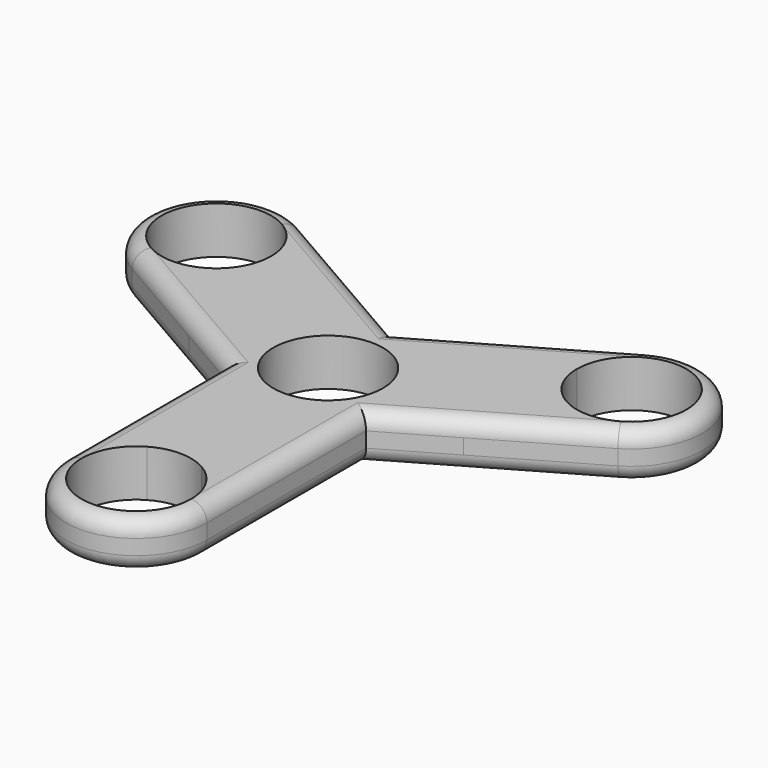
from build123d import *

# Parameters (mm, degrees)
F0_R          = 3.5
F1_DEPTH      = 3
F2_T4_DEPTH   = 15.24
F2_T9_DEPTH   = 15.24
F2_T14_DEPTH  = 15.24
F2_T19_DEPTH  = 15.24
F2_T24_DEPTH  = 15.24
F2_T29_DEPTH  = 15.24
F2_T32_ANGLE  = 180
F2_T34_ANGLE  = 180
F2_T36_ANGLE  = 180
F2_T40_DEPTH  = 15.24
F2_T45_DEPTH  = 15.24
F2_T50_DEPTH  = 15.24
F2_T55_DEPTH  = 15.24
F2_T58_ANGLE  = 180
F2_T62_DEPTH  = 15.24
F2_T65_ANGLE  = 180
F2_T67_ANGLE  = 180
F2_T71_DEPTH  = 15.24
F2_T77_DEPTH  = 15.24
F2_T81_DEPTH  = 15.24
F2_T88_DEPTH  = 15.24
F2_T92_DEPTH  = 15.24
F2_T99_DEPTH  = 15.24
F2_T103_DEPTH = 15.24
F2_T110_DEPTH = 15.24
F2_T114_DEPTH = 15.24
F2_T121_DEPTH = 15.24
F2_T125_DEPTH = 15.24
F2_T132_DEPTH = 15.24
F2_T136_DEPTH = 15.24


# Not quite as in the source:
# - a fillet or chamfer that OpenCascade refuses, or shapes differently, is made with other operations: its cross-section is extruded or revolved along the edge and cut away or added


with BuildPart() as f1:
    # F0 (on Top) → F1 (new body)
    with BuildSketch(Plane.XY):
        with BuildLine():
            Line((-9.7485226281, 10.247114317), (-8.7485226281, 10.247114317))
            ThreePointArc((-8.7485226281, 10.247114317), (-9.351408311, 12.497114317), (-10.9985226281, 14.1442286341))
            ThreePointArc((-10.9985226281, 14.1442286341), (-17.1456369451, 12.497114317), (-15.4985226281, 6.35))
            ThreePointArc((-15.4985226281, 6.35), (-13.2485226281, 5.747114317), (-10.9985226281, 6.35))
            Line((-10.9985226281, 6.35), (-11.4985226281, 7.2160254038))
            ThreePointArc((-11.4985226281, 7.2160254038), (-16.2796115413, 11.997114317), (-9.7485226281, 10.247114317))
        make_face()
        with BuildLine():
            ThreePointArc((-10.9985226281, 6.35), (-9.351408311, 7.997114317), (-8.7485226281, 10.247114317))
            Line((-8.7485226281, 10.247114317), (-9.7485226281, 10.247114317))
            ThreePointArc((-9.7485226281, 10.247114317), (-10.2174337148, 8.497114317), (-11.4985226281, 7.2160254038))
            Line((-11.4985226281, 7.2160254038), (-10.9985226281, 6.35))
        make_face()
        with BuildLine():
            Line((9.7485226281, 10.247114317), (8.7485226281, 10.247114317))
            ThreePointArc((8.7485226281, 10.247114317), (9.351408311, 7.997114317), (10.9985226281, 6.35))
            Line((10.9985226281, 6.35), (11.4985226281, 7.2160254038))
            ThreePointArc((11.4985226281, 7.2160254038), (10.2174337148, 8.497114317), (9.7485226281, 10.247114317))
        make_face()
        with BuildLine():
            ThreePointArc((17.7485226281, 10.247114317), (15.4985226281, 14.1442286341), (10.9985226281, 14.1442286341))
            ThreePointArc((10.9985226281, 14.1442286341), (9.351408311, 12.497114317), (8.7485226281, 10.247114317))
            Line((8.7485226281, 10.247114317), (9.7485226281, 10.247114317))
            ThreePointArc((9.7485226281, 10.247114317), (13.2485226281, 13.747114317), (16.7485226281, 10.247114317))
            ThreePointArc((16.7485226281, 10.247114317), (14.9985226281, 7.2160254038), (11.4985226281, 7.2160254038))
            Line((11.4985226281, 7.2160254038), (10.9985226281, 6.35))
            ThreePointArc((10.9985226281, 6.35), (13.2485226281, 5.747114317), (15.4985226281, 6.35))
            ThreePointArc((15.4985226281, 6.35), (17.1456369451, 7.997114317), (17.7485226281, 10.247114317))
        make_face()
        with BuildLine():
            ThreePointArc((2.25, -8.802885683), (0, -8.2), (-2.25, -8.802885683))
            Line((-2.25, -8.802885683), (-1.75, -9.6689110868))
            ThreePointArc((-1.75, -9.6689110868), (0, -9.2), (1.75, -9.6689110868))
            Line((1.75, -9.6689110868), (2.25, -8.802885683))
        make_face()
        with BuildLine():
            ThreePointArc((-2.25, -8.802885683), (-3.897114317, -10.45), (-4.5, -12.7))
            ThreePointArc((-4.5, -12.7), (0, -17.2), (4.5, -12.7))
            ThreePointArc((4.5, -12.7), (3.897114317, -10.45), (2.25, -8.802885683))
            Line((2.25, -8.802885683), (1.75, -9.6689110868))
            ThreePointArc((1.75, -9.6689110868), (3.0310889132, -10.95), (3.5, -12.7))
            ThreePointArc((3.5, -12.7), (-1.75, -15.7310889132), (-1.75, -9.6689110868))
            Line((-1.75, -9.6689110868), (-2.25, -8.802885683))
        make_face()
        with BuildLine():
            Line((-4.2485226281, 10.247114317), (-8.7485226281, 10.247114317))
            ThreePointArc((-8.7485226281, 10.247114317), (-9.351408311, 7.997114317), (-10.9985226281, 6.35))
            Line((-10.9985226281, 6.35), (-8.7485226281, 2.452885683))
            Line((-8.7485226281, 2.452885683), (-4.5, 0))
            Line((-4.5, 0), (-4.5, -4.9057713659))
            Line((-4.5, -4.9057713659), (-2.25, -8.802885683))
            ThreePointArc((-2.25, -8.802885683), (0, -8.2), (2.25, -8.802885683))
            Line((2.25, -8.802885683), (4.5, -4.9057713659))
            Line((4.5, -4.9057713659), (4.5, 0))
            Line((4.5, 0), (8.7485226281, 2.452885683))
            Line((8.7485226281, 2.452885683), (10.9985226281, 6.35))
            ThreePointArc((10.9985226281, 6.35), (9.351408311, 7.997114317), (8.7485226281, 10.247114317))
            Line((8.7485226281, 10.247114317), (4.2485226281, 10.247114317))
            Line((4.2485226281, 10.247114317), (0, 7.7942286341))
            Line((0, 7.7942286341), (-4.2485226281, 10.247114317))
        make_face()
        with Locations((0, 2.5980762114)):
            Circle(F0_R, mode=Mode.SUBTRACT)
        with BuildLine():
            Line((-2.25, -8.802885683), (-4.5, -4.9057713659))
            Line((-4.5, -4.9057713659), (-4.5, -12.7))
            ThreePointArc((-4.5, -12.7), (-3.897114317, -10.45), (-2.25, -8.802885683))
        make_face()
        with BuildLine():
            ThreePointArc((2.25, -8.802885683), (3.897114317, -10.45), (4.5, -12.7))
            Line((4.5, -12.7), (4.5, -4.9057713659))
            Line((4.5, -4.9057713659), (2.25, -8.802885683))
        make_face()
        with BuildLine():
            ThreePointArc((15.4985226281, 6.35), (13.2485226281, 5.747114317), (10.9985226281, 6.35))
            Line((10.9985226281, 6.35), (8.7485226281, 2.452885683))
            Line((8.7485226281, 2.452885683), (15.4985226281, 6.35))
        make_face()
        with BuildLine():
            Line((10.9985226281, 14.1442286341), (4.2485226281, 10.247114317))
            Line((4.2485226281, 10.247114317), (8.7485226281, 10.247114317))
            ThreePointArc((8.7485226281, 10.247114317), (9.351408311, 12.497114317), (10.9985226281, 14.1442286341))
        make_face()
        with BuildLine():
            ThreePointArc((-10.9985226281, 14.1442286341), (-9.351408311, 12.497114317), (-8.7485226281, 10.247114317))
            Line((-8.7485226281, 10.247114317), (-4.2485226281, 10.247114317))
            Line((-4.2485226281, 10.247114317), (-10.9985226281, 14.1442286341))
        make_face()
        with BuildLine():
            Line((-8.7485226281, 2.452885683), (-10.9985226281, 6.35))
            ThreePointArc((-10.9985226281, 6.35), (-13.2485226281, 5.747114317), (-15.4985226281, 6.35))
            Line((-15.4985226281, 6.35), (-8.7485226281, 2.452885683))
        make_face()
    extrude(amount=F1_DEPTH)

    # F2: fillet of radius 1.016 on 18 edges, made by hand


with BuildPart() as f2_tool2:
    # F2_s3 → F2_t4 (new body)
    with BuildSketch(Plane(origin=(14.3735226281, 8.2985571585, 0), x_dir=(0, 0, 1), z_dir=(-0.8660254038, -0.5, 0))):
        with BuildLine():
            ThreePointArc((1.984, 6.75), (2.7024204897, 6.4524204897), (3, 5.734))
            Line((3, 5.734), (3, 6.75))
            Line((3, 6.75), (1.984, 6.75))
        make_face()
    extrude(amount=F2_T4_DEPTH)

    split(bisect_by=Plane(origin=(3.375, 5.8456714755, 0), x_dir=(0, 0, 1), z_dir=(0.5, 0.8660254038, 0)), keep=Keep.TOP)


with BuildPart() as f1_1:
    add(f1.part)

    # F2_t1: cut F2_tool2
    add(f2_tool2.part, mode=Mode.SUBTRACT)


with BuildPart() as f2_tool7:
    # F2_s8 → F2_t9 (new body)
    with BuildSketch(Plane(origin=(1.1752954744, 0.6785571585, 0), x_dir=(0, 0, 1), z_dir=(0.8660254038, 0.5, 0))):
        with BuildLine():
            ThreePointArc((1.984, 2.25), (2.7024204897, 1.9524204897), (3, 1.234))
            Line((3, 1.234), (3, 2.25))
            Line((3, 2.25), (1.984, 2.25))
        make_face()
    extrude(amount=F2_T9_DEPTH)

    split(bisect_by=Plane.YZ.offset(4.5), keep=Keep.TOP)


with BuildPart() as f1_2:
    add(f1_1.part)

    # F2_t6: cut F2_tool7
    add(f2_tool7.part, mode=Mode.SUBTRACT)


with BuildPart() as f2_tool12:
    # F2_s13 → F2_t14 (new body)
    with BuildSketch(Plane(origin=(-1.1752954744, 0.6785571585, 0), x_dir=(0, 0, 1), z_dir=(-0.8660254038, 0.5, 0))):
        with BuildLine():
            ThreePointArc((1.984, 6.75), (2.7024204897, 6.4524204897), (3, 5.734))
            Line((3, 5.734), (3, 6.75))
            Line((3, 6.75), (1.984, 6.75))
        make_face()
    extrude(amount=F2_T14_DEPTH)

    split(bisect_by=Plane(origin=(-3.375, 5.8456714755, 0), x_dir=(0, 0, 1), z_dir=(-0.5, 0.8660254038, 0)), keep=Keep.TOP)


with BuildPart() as f1_3:
    add(f1_2.part)

    # F2_t11: cut F2_tool12
    add(f2_tool12.part, mode=Mode.SUBTRACT)


with BuildPart() as f2_tool17:
    # F2_s18 → F2_t19 (new body)
    with BuildSketch(Plane(origin=(-14.3735226281, 8.2985571585, 0), x_dir=(0, 0, 1), z_dir=(0.8660254038, -0.5, 0))):
        with BuildLine():
            ThreePointArc((1.984, 2.25), (2.7024204897, 1.9524204897), (3, 1.234))
            Line((3, 1.234), (3, 2.25))
            Line((3, 2.25), (1.984, 2.25))
        make_face()
    extrude(amount=F2_T19_DEPTH)

    split(bisect_by=Plane.YZ.offset(-4.5), keep=Keep.BOTTOM)


with BuildPart() as f1_4:
    add(f1_3.part)

    # F2_t16: cut F2_tool17
    add(f2_tool17.part, mode=Mode.SUBTRACT)


with BuildPart() as f2_tool22:
    # F2_s23 → F2_t24 (new body)
    with BuildSketch(Plane.XZ.offset(-2.54)):
        with BuildLine():
            ThreePointArc((-4.5, 1.984), (-4.2024204897, 2.7024204897), (-3.484, 3))
            Line((-3.484, 3), (-4.5, 3))
            Line((-4.5, 3), (-4.5, 1.984))
        make_face()
    extrude(amount=F2_T24_DEPTH)

    split(bisect_by=Plane(origin=(-1.125, -1.9485571585, 0), x_dir=(0, 0, 1), z_dir=(-0.5, -0.8660254038, 0)), keep=Keep.TOP)


with BuildPart() as f1_5:
    add(f1_4.part)

    # F2_t21: cut F2_tool22
    add(f2_tool22.part, mode=Mode.SUBTRACT)


with BuildPart() as f2_tool27:
    # F2_s28 → F2_t29 (new body)
    with BuildSketch(Plane.XZ.offset(12.7)):
        with BuildLine():
            ThreePointArc((4.5, 1.984), (4.2024204897, 2.7024204897), (3.484, 3))
            Line((3.484, 3), (4.5, 3))
            Line((4.5, 3), (4.5, 1.984))
        make_face()
    extrude(amount=-F2_T29_DEPTH)

    split(bisect_by=Plane(origin=(1.125, -1.9485571585, 0), x_dir=(0, 0, 1), z_dir=(0.5, -0.8660254038, 0)), keep=Keep.TOP)


with BuildPart() as f1_6:
    add(f1_5.part)

    # F2_t26: cut F2_tool27
    add(f2_tool27.part, mode=Mode.SUBTRACT)

    # F2_s31 → F2_t32 (revolve, cut)
    with BuildSketch(Plane.XZ.offset(12.7)):
        with BuildLine():
            ThreePointArc((-4.5, 1.984), (-4.2024204897, 2.7024204897), (-3.484, 3))
            Line((-3.484, 3), (-4.5, 3))
            Line((-4.5, 3), (-4.5, 1.984))
        make_face()
    revolve(axis=Axis((0, -12.7, 3), (0, 0, 1)), revolution_arc=F2_T32_ANGLE, mode=Mode.SUBTRACT)

    # F2_s33 → F2_t34 (revolve, cut)
    with BuildSketch(Plane(origin=(-14.3735226281, 8.2985571585, 0), x_dir=(0, 0, 1), z_dir=(0.8660254038, -0.5, 0))):
        with BuildLine():
            ThreePointArc((1.984, -6.75), (2.7024204897, -6.4524204897), (3, -5.734))
            Line((3, -5.734), (3, -6.75))
            Line((3, -6.75), (1.984, -6.75))
        make_face()
    revolve(axis=Axis((-13.2485226281, 10.247114317, 3), (0, 0, 1)), revolution_arc=F2_T34_ANGLE, mode=Mode.SUBTRACT)

    # F2_s35 → F2_t36 (revolve, cut)
    with BuildSketch(Plane(origin=(14.3735226281, 8.2985571585, 0), x_dir=(0, 0, 1), z_dir=(-0.8660254038, -0.5, 0))):
        with BuildLine():
            ThreePointArc((1.984, -2.25), (2.7024204897, -1.9524204897), (3, -1.234))
            Line((3, -1.234), (3, -2.25))
            Line((3, -2.25), (1.984, -2.25))
        make_face()
    revolve(axis=Axis((13.2485226281, 10.247114317, 3), (0, 0, 1)), revolution_arc=F2_T36_ANGLE, mode=Mode.SUBTRACT)


with BuildPart() as f2_tool38:
    # F2_s39 → F2_t40 (new body)
    with BuildSketch(Plane(origin=(-14.3735226281, 8.2985571585, 0), x_dir=(0, 0, 1), z_dir=(0.8660254038, -0.5, 0))):
        with BuildLine():
            ThreePointArc((1.016, 2.25), (0.2975795103, 1.9524204897), (0, 1.234))
            Line((0, 1.234), (0, 2.25))
            Line((0, 2.25), (1.016, 2.25))
        make_face()
    extrude(amount=F2_T40_DEPTH)

    split(bisect_by=Plane.YZ.offset(-4.5), keep=Keep.BOTTOM)


with BuildPart() as f1_7:
    add(f1_6.part)

    # F2_t37: cut F2_tool38
    add(f2_tool38.part, mode=Mode.SUBTRACT)


with BuildPart() as f2_tool43:
    # F2_s44 → F2_t45 (new body)
    with BuildSketch(Plane.XZ.offset(-2.54)):
        with BuildLine():
            ThreePointArc((-4.5, 1.016), (-4.2024204897, 0.2975795103), (-3.484, 0))
            Line((-3.484, 0), (-4.5, 0))
            Line((-4.5, 0), (-4.5, 1.016))
        make_face()
    extrude(amount=F2_T45_DEPTH)

    split(bisect_by=Plane(origin=(-1.125, -1.9485571585, 0), x_dir=(0, 0, 1), z_dir=(-0.5, -0.8660254038, 0)), keep=Keep.TOP)


with BuildPart() as f1_8:
    add(f1_7.part)

    # F2_t42: cut F2_tool43
    add(f2_tool43.part, mode=Mode.SUBTRACT)


with BuildPart() as f2_tool48:
    # F2_s49 → F2_t50 (new body)
    with BuildSketch(Plane.XZ.offset(12.7)):
        with BuildLine():
            ThreePointArc((4.5, 1.016), (4.2024204897, 0.2975795103), (3.484, 0))
            Line((3.484, 0), (4.5, 0))
            Line((4.5, 0), (4.5, 1.016))
        make_face()
    extrude(amount=-F2_T50_DEPTH)

    split(bisect_by=Plane(origin=(1.125, -1.9485571585, 0), x_dir=(0, 0, 1), z_dir=(0.5, -0.8660254038, 0)), keep=Keep.TOP)


with BuildPart() as f1_9:
    add(f1_8.part)

    # F2_t47: cut F2_tool48
    add(f2_tool48.part, mode=Mode.SUBTRACT)


with BuildPart() as f2_tool53:
    # F2_s54 → F2_t55 (new body)
    with BuildSketch(Plane(origin=(1.1752954744, 0.6785571585, 0), x_dir=(0, 0, 1), z_dir=(0.8660254038, 0.5, 0))):
        with BuildLine():
            ThreePointArc((1.016, 2.25), (0.2975795103, 1.9524204897), (0, 1.234))
            Line((0, 1.234), (0, 2.25))
            Line((0, 2.25), (1.016, 2.25))
        make_face()
    extrude(amount=F2_T55_DEPTH)

    split(bisect_by=Plane.YZ.offset(4.5), keep=Keep.TOP)


with BuildPart() as f1_10:
    add(f1_9.part)

    # F2_t52: cut F2_tool53
    add(f2_tool53.part, mode=Mode.SUBTRACT)

    # F2_s57 → F2_t58 (revolve, cut)
    with BuildSketch(Plane(origin=(14.3735226281, 8.2985571585, 0), x_dir=(0, 0, 1), z_dir=(-0.8660254038, -0.5, 0))):
        with BuildLine():
            ThreePointArc((1.016, -2.25), (0.2975795103, -1.9524204897), (0, -1.234))
            Line((0, -1.234), (0, -2.25))
            Line((0, -2.25), (1.016, -2.25))
        make_face()
    revolve(axis=Axis((13.2485226281, 10.247114317, 0), (0, 0, 1)), revolution_arc=F2_T58_ANGLE, mode=Mode.SUBTRACT)


with BuildPart() as f2_tool60:
    # F2_s61 → F2_t62 (new body)
    with BuildSketch(Plane(origin=(14.3735226281, 8.2985571585, 0), x_dir=(0, 0, 1), z_dir=(-0.8660254038, -0.5, 0))):
        with BuildLine():
            ThreePointArc((1.016, 6.75), (0.2975795103, 6.4524204897), (0, 5.734))
            Line((0, 5.734), (0, 6.75))
            Line((0, 6.75), (1.016, 6.75))
        make_face()
    extrude(amount=F2_T62_DEPTH)

    split(bisect_by=Plane(origin=(3.375, 5.8456714755, 0), x_dir=(0, 0, 1), z_dir=(0.5, 0.8660254038, 0)), keep=Keep.TOP)


with BuildPart() as f1_11:
    add(f1_10.part)

    # F2_t59: cut F2_tool60
    add(f2_tool60.part, mode=Mode.SUBTRACT)

    # F2_s64 → F2_t65 (revolve, cut)
    with BuildSketch(Plane.XZ.offset(12.7)):
        with BuildLine():
            ThreePointArc((-4.5, 1.016), (-4.2024204897, 0.2975795103), (-3.484, 0))
            Line((-3.484, 0), (-4.5, 0))
            Line((-4.5, 0), (-4.5, 1.016))
        make_face()
    revolve(axis=Axis((0, -12.7, 0), (0, 0, 1)), revolution_arc=F2_T65_ANGLE, mode=Mode.SUBTRACT)

    # F2_s66 → F2_t67 (revolve, cut)
    with BuildSketch(Plane(origin=(-14.3735226281, 8.2985571585, 0), x_dir=(0, 0, 1), z_dir=(0.8660254038, -0.5, 0))):
        with BuildLine():
            ThreePointArc((1.016, -6.75), (0.2975795103, -6.4524204897), (0, -5.734))
            Line((0, -5.734), (0, -6.75))
            Line((0, -6.75), (1.016, -6.75))
        make_face()
    revolve(axis=Axis((-13.2485226281, 10.247114317, 0), (0, 0, 1)), revolution_arc=F2_T67_ANGLE, mode=Mode.SUBTRACT)


with BuildPart() as f2_tool69:
    # F2_s70 → F2_t71 (new body)
    with BuildSketch(Plane(origin=(-1.1752954744, 0.6785571585, 0), x_dir=(0, 0, 1), z_dir=(-0.8660254038, 0.5, 0))):
        with BuildLine():
            ThreePointArc((1.016, 6.75), (0.2975795103, 6.4524204897), (0, 5.734))
            Line((0, 5.734), (0, 6.75))
            Line((0, 6.75), (1.016, 6.75))
        make_face()
    extrude(amount=F2_T71_DEPTH)

    split(bisect_by=Plane(origin=(-3.375, 5.8456714755, 0), x_dir=(0, 0, 1), z_dir=(-0.5, 0.8660254038, 0)), keep=Keep.TOP)


with BuildPart() as f1_12:
    add(f1_11.part)

    # F2_t68: cut F2_tool69
    add(f2_tool69.part, mode=Mode.SUBTRACT)


with BuildPart() as f2_tool75:
    # F2_s76 → F2_t77 (new body)
    with BuildSketch(Plane(origin=(14.3735226281, 8.2985571585, 0), x_dir=(0, 0, 1), z_dir=(-0.8660254038, -0.5, 0))):
        with BuildLine():
            ThreePointArc((1.984, 6.75), (2.7024204897, 6.4524204897), (3, 5.734))
            Line((3, 5.734), (3, 6.75))
            Line((3, 6.75), (1.984, 6.75))
        make_face()
    extrude(amount=F2_T77_DEPTH)

    split(bisect_by=Plane(origin=(3.375, 5.8456714755, 0), x_dir=(0, 0, 1), z_dir=(-0.5, -0.8660254038, 0)), keep=Keep.TOP)


with BuildPart() as f2_tool79:
    # F2_s80 → F2_t81 (new body)
    with BuildSketch(Plane(origin=(-1.1752954744, 0.6785571585, 0), x_dir=(0, 0, 1), z_dir=(-0.8660254038, 0.5, 0))):
        with BuildLine():
            ThreePointArc((1.984, 6.75), (2.7024204897, 6.4524204897), (3, 5.734))
            Line((3, 5.734), (3, 6.75))
            Line((3, 6.75), (1.984, 6.75))
        make_face()
    extrude(amount=F2_T81_DEPTH)

    split(bisect_by=Plane(origin=(-3.375, 5.8456714755, 0), x_dir=(0, 0, 1), z_dir=(0.5, -0.8660254038, 0)), keep=Keep.TOP)


with BuildPart() as f2_tool75_1:
    add(f2_tool75.part)

    # F2_t83: intersect F2_tool79
    add(f2_tool79.part, mode=Mode.INTERSECT)


with BuildPart() as f1_13:
    add(f1_12.part)

    # F2_t73: cut F2_tool75
    add(f2_tool75_1.part, mode=Mode.SUBTRACT)


with BuildPart() as f2_tool86:
    # F2_s87 → F2_t88 (new body)
    with BuildSketch(Plane.XZ.offset(12.7)):
        with BuildLine():
            ThreePointArc((4.5, 1.984), (4.2024204897, 2.7024204897), (3.484, 3))
            Line((3.484, 3), (4.5, 3))
            Line((4.5, 3), (4.5, 1.984))
        make_face()
    extrude(amount=-F2_T88_DEPTH)

    split(bisect_by=Plane(origin=(1.125, -1.9485571585, 0), x_dir=(0, 0, 1), z_dir=(-0.5, 0.8660254038, 0)), keep=Keep.TOP)


with BuildPart() as f2_tool90:
    # F2_s91 → F2_t92 (new body)
    with BuildSketch(Plane(origin=(1.1752954744, 0.6785571585, 0), x_dir=(0, 0, 1), z_dir=(0.8660254038, 0.5, 0))):
        with BuildLine():
            ThreePointArc((1.984, 2.25), (2.7024204897, 1.9524204897), (3, 1.234))
            Line((3, 1.234), (3, 2.25))
            Line((3, 2.25), (1.984, 2.25))
        make_face()
    extrude(amount=F2_T92_DEPTH)

    split(bisect_by=Plane.YZ.offset(4.5), keep=Keep.BOTTOM)


with BuildPart() as f2_tool86_1:
    add(f2_tool86.part)

    # F2_t94: intersect F2_tool90
    add(f2_tool90.part, mode=Mode.INTERSECT)


with BuildPart() as f1_14:
    add(f1_13.part)

    # F2_t84: cut F2_tool86
    add(f2_tool86_1.part, mode=Mode.SUBTRACT)


with BuildPart() as f2_tool97:
    # F2_s98 → F2_t99 (new body)
    with BuildSketch(Plane(origin=(-14.3735226281, 8.2985571585, 0), x_dir=(0, 0, 1), z_dir=(0.8660254038, -0.5, 0))):
        with BuildLine():
            ThreePointArc((1.984, 2.25), (2.7024204897, 1.9524204897), (3, 1.234))
            Line((3, 1.234), (3, 2.25))
            Line((3, 2.25), (1.984, 2.25))
        make_face()
    extrude(amount=F2_T99_DEPTH)

    split(bisect_by=Plane.YZ.offset(-4.5), keep=Keep.TOP)


with BuildPart() as f2_tool101:
    # F2_s102 → F2_t103 (new body)
    with BuildSketch(Plane.XZ.offset(-2.54)):
        with BuildLine():
            ThreePointArc((-4.5, 1.984), (-4.2024204897, 2.7024204897), (-3.484, 3))
            Line((-3.484, 3), (-4.5, 3))
            Line((-4.5, 3), (-4.5, 1.984))
        make_face()
    extrude(amount=F2_T103_DEPTH)

    split(bisect_by=Plane(origin=(-1.125, -1.9485571585, 0), x_dir=(0, 0, 1), z_dir=(0.5, 0.8660254038, 0)), keep=Keep.TOP)


with BuildPart() as f2_tool97_1:
    add(f2_tool97.part)

    # F2_t105: intersect F2_tool101
    add(f2_tool101.part, mode=Mode.INTERSECT)


with BuildPart() as f1_15:
    add(f1_14.part)

    # F2_t95: cut F2_tool97
    add(f2_tool97_1.part, mode=Mode.SUBTRACT)


with BuildPart() as f2_tool108:
    # F2_s109 → F2_t110 (new body)
    with BuildSketch(Plane(origin=(-14.3735226281, 8.2985571585, 0), x_dir=(0, 0, 1), z_dir=(0.8660254038, -0.5, 0))):
        with BuildLine():
            ThreePointArc((1.016, 2.25), (0.2975795103, 1.9524204897), (0, 1.234))
            Line((0, 1.234), (0, 2.25))
            Line((0, 2.25), (1.016, 2.25))
        make_face()
    extrude(amount=F2_T110_DEPTH)

    split(bisect_by=Plane.YZ.offset(-4.5), keep=Keep.TOP)


with BuildPart() as f2_tool112:
    # F2_s113 → F2_t114 (new body)
    with BuildSketch(Plane.XZ.offset(-2.54)):
        with BuildLine():
            ThreePointArc((-4.5, 1.016), (-4.2024204897, 0.2975795103), (-3.484, 0))
            Line((-3.484, 0), (-4.5, 0))
            Line((-4.5, 0), (-4.5, 1.016))
        make_face()
    extrude(amount=F2_T114_DEPTH)

    split(bisect_by=Plane(origin=(-1.125, -1.9485571585, 0), x_dir=(0, 0, 1), z_dir=(0.5, 0.8660254038, 0)), keep=Keep.TOP)


with BuildPart() as f2_tool108_1:
    add(f2_tool108.part)

    # F2_t116: intersect F2_tool112
    add(f2_tool112.part, mode=Mode.INTERSECT)


with BuildPart() as f1_16:
    add(f1_15.part)

    # F2_t106: cut F2_tool108
    add(f2_tool108_1.part, mode=Mode.SUBTRACT)


with BuildPart() as f2_tool119:
    # F2_s120 → F2_t121 (new body)
    with BuildSketch(Plane.XZ.offset(12.7)):
        with BuildLine():
            ThreePointArc((4.5, 1.016), (4.2024204897, 0.2975795103), (3.484, 0))
            Line((3.484, 0), (4.5, 0))
            Line((4.5, 0), (4.5, 1.016))
        make_face()
    extrude(amount=-F2_T121_DEPTH)

    split(bisect_by=Plane(origin=(1.125, -1.9485571585, 0), x_dir=(0, 0, 1), z_dir=(-0.5, 0.8660254038, 0)), keep=Keep.TOP)


with BuildPart() as f2_tool123:
    # F2_s124 → F2_t125 (new body)
    with BuildSketch(Plane(origin=(1.1752954744, 0.6785571585, 0), x_dir=(0, 0, 1), z_dir=(0.8660254038, 0.5, 0))):
        with BuildLine():
            ThreePointArc((1.016, 2.25), (0.2975795103, 1.9524204897), (0, 1.234))
            Line((0, 1.234), (0, 2.25))
            Line((0, 2.25), (1.016, 2.25))
        make_face()
    extrude(amount=F2_T125_DEPTH)

    split(bisect_by=Plane.YZ.offset(4.5), keep=Keep.BOTTOM)


with BuildPart() as f2_tool119_1:
    add(f2_tool119.part)

    # F2_t127: intersect F2_tool123
    add(f2_tool123.part, mode=Mode.INTERSECT)


with BuildPart() as f1_17:
    add(f1_16.part)

    # F2_t117: cut F2_tool119
    add(f2_tool119_1.part, mode=Mode.SUBTRACT)


with BuildPart() as f2_tool130:
    # F2_s131 → F2_t132 (new body)
    with BuildSketch(Plane(origin=(14.3735226281, 8.2985571585, 0), x_dir=(0, 0, 1), z_dir=(-0.8660254038, -0.5, 0))):
        with BuildLine():
            ThreePointArc((1.016, 6.75), (0.2975795103, 6.4524204897), (0, 5.734))
            Line((0, 5.734), (0, 6.75))
            Line((0, 6.75), (1.016, 6.75))
        make_face()
    extrude(amount=F2_T132_DEPTH)

    split(bisect_by=Plane(origin=(3.375, 5.8456714755, 0), x_dir=(0, 0, 1), z_dir=(-0.5, -0.8660254038, 0)), keep=Keep.TOP)


with BuildPart() as f2_tool134:
    # F2_s135 → F2_t136 (new body)
    with BuildSketch(Plane(origin=(-1.1752954744, 0.6785571585, 0), x_dir=(0, 0, 1), z_dir=(-0.8660254038, 0.5, 0))):
        with BuildLine():
            ThreePointArc((1.016, 6.75), (0.2975795103, 6.4524204897), (0, 5.734))
            Line((0, 5.734), (0, 6.75))
            Line((0, 6.75), (1.016, 6.75))
        make_face()
    extrude(amount=F2_T136_DEPTH)

    split(bisect_by=Plane(origin=(-3.375, 5.8456714755, 0), x_dir=(0, 0, 1), z_dir=(0.5, -0.8660254038, 0)), keep=Keep.TOP)


with BuildPart() as f2_tool130_1:
    add(f2_tool130.part)

    # F2_t138: intersect F2_tool134
    add(f2_tool134.part, mode=Mode.INTERSECT)


with BuildPart() as f1_18:
    add(f1_17.part)

    # F2_t128: cut F2_tool130
    add(f2_tool130_1.part, mode=Mode.SUBTRACT)


solid = f1_18.part
